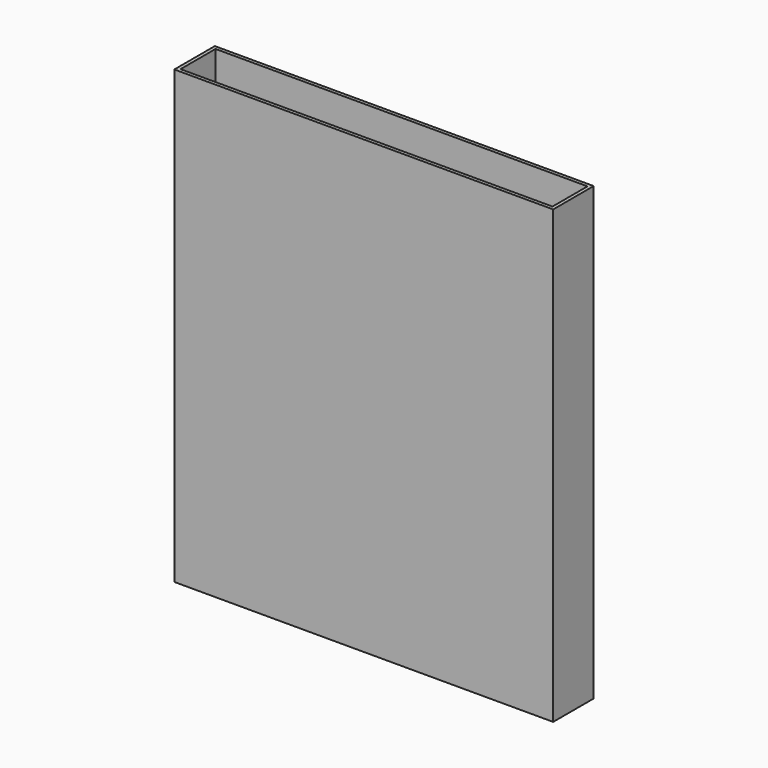
from build123d import *

# Parameters (mm, degrees)
F0_W     = 54
F0_H     = 6.35
F1_DEPTH = 65
F2_T     = 0.5


with BuildPart() as f1:
    # F0 (on Top) → F1 (new body)
    with BuildSketch(Plane.XY):
        Rectangle(F0_W, F0_H)
    extrude(amount=F1_DEPTH)

    # F2
    f2_openings = [f1.faces().sort_by_distance(p)[0] for p in [
        (0, 0, 65),
    ]]
    offset(amount=F2_T, openings=f2_openings, kind=Kind.INTERSECTION)


solid = f1.part
